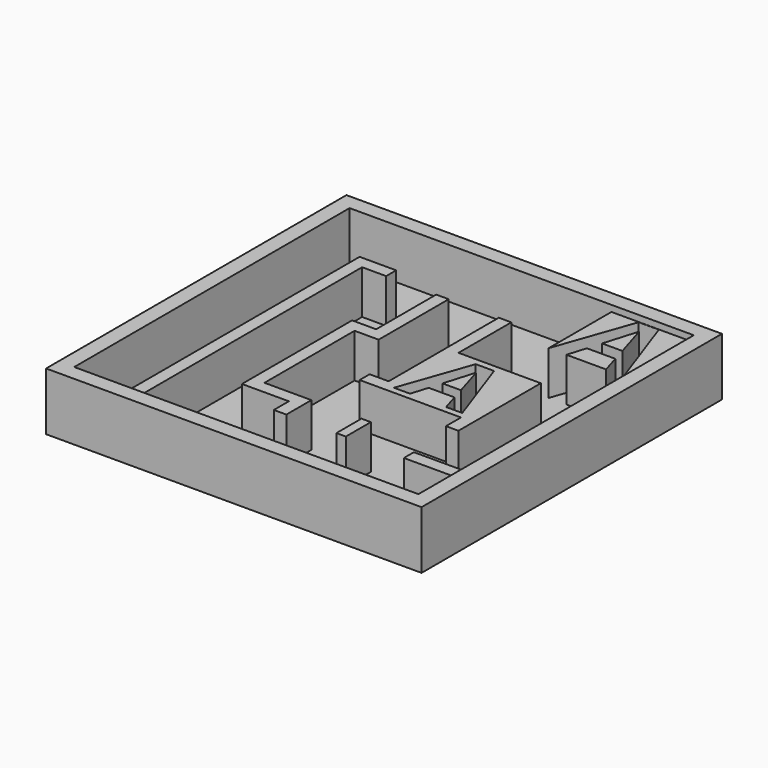
from build123d import *

# Parameters (mm, degrees)
F0_W         = 38.1
F0_H         = 38.1
F1_DEPTH     = 0.79375
F2_W         = 38.1
F2_H         = 38.1
F2_W_2       = 34.925
F2_H_2       = 34.925
F3_DEPTH     = 5.08
F4_W         = 5.5410787107
F4_H         = 1.27
F4_TEXT_SIZE = 11.0670119076
F4_W_2       = 0.9547267341
F4_H_2       = 3.175
F5_DEPTH     = 4.445
F7_DEPTH     = 25.4
F6_R         = 1.27
F6_TEXT_SIZE = 10.0575314688
F8_DEPTH     = 4.445
F9_DEPTH     = 4.445
F10_DEPTH    = 0.396875
F11_DEPTH    = 0.396875


# Not quite as in the source:
# - Text() gives the source's letters only with a copy of the font that has no kerning and outlines rounded to 1/6400 em; it was checked with that copy


with BuildPart() as f1:
    # F0 (on Top) → F1 (new body)
    with BuildSketch(Plane.XY):
        with Locations((0.2368067951, -2.7494172126)):
            Rectangle(F0_W, F0_H)
    extrude(amount=F1_DEPTH)

    # F2 (on face) → F3 (join)
    with BuildSketch(Plane.XY.offset(0.79375)):
        with Locations((0.2368067951, -2.7494172126)):
            Rectangle(F2_W, F2_H)
        with Locations((0.2368067951, -2.7494172126)):
            Rectangle(F2_W_2, F2_H_2, mode=Mode.SUBTRACT)
    extrude(amount=F3_DEPTH)

    # F4 (on face) → F5 (join)
    with BuildSketch(Plane.XY.offset(0.79375)):
        Polygon((-12.1456932049, 9.6330827874), (-12.1456932049, -20.2119172126), (-10.8756932049, -20.2119172126), (-10.8756932049, 8.3630827874), (-8.4345579745, 8.3630827874), (-8.4345579745, 9.6330827874), (-10.8756932049, 9.6330827874), align=None)
        with Locations((14.9287674398, -14.4969172126)):
            Rectangle(F4_W, F4_H)
        Polygon((17.6993067951, 14.7130827874), (9.3454420255, 14.7130827874), (9.3454420255, 6.7448342139), (12.1346748703, 14.6784983752), (14.1820720732, 14.6784983752), (16.9816802417, 6.7448342139), (17.6993067951, 6.7448342139), align=None)
        with Locations((9.3454420255, 6.7448342139)):
            Text('A', F4_TEXT_SIZE, font='Open Sans', font_style=FontStyle.BOLD, text_align=(TextAlign.LEFT, TextAlign.BOTTOM))
        Polygon((11.723120365, 8.6262262382), (11.1507483429, 6.7448342139), (15.1763739243, 6.7448342139), (14.6040019022, 8.6262262382), align=None)
        Polygon((-2.0845579745, 8.3630827874), (-3.3545579745, 8.3630827874), (-3.3545579745, 0.7430827874), (-5.7956932049, 0.7430827874), (-5.7956932049, -0.5269172126), (-5.7956932049, -13.2269172126), (-4.5256932049, -13.2269172126), (-1.035419939, -13.2269172126), (-1.035419939, -15.1319172126), (0.234580061, -15.1319172126), (0.234580061, -13.2269172126), (0.234580061, -11.9569172126), (-4.5256932049, -11.9569172126), (-4.5256932049, -0.5269172126), (-2.0845579745, -0.5269172126), (-2.0845579745, 0.7430827874), align=None)
        Polygon((4.2654420255, 8.3630827874), (2.9954420255, 8.3630827874), (2.9954420255, 4.3662126074), (2.9954420255, 1.6648342139), (2.9954420255, -5.6069172126), (1.0636646766, -5.6069172126), (1.0636646766, -6.8769172126), (2.9954420255, -6.8769172126), (6.2693067951, -6.8769172126), (11.3493067951, -6.8769172126), (11.3493067951, -8.7819172126), (12.6193067951, -8.7819172126), (12.6193067951, -6.8769172126), (12.6193067951, -6.8514254262), (12.6193067951, 1.6648342139), (4.2654420255, 1.6648342139), align=None)
        with Locations((5.7919434281, -13.5444172126)):
            Rectangle(F4_W_2, F4_H_2)
        with BuildLine():
            Line((12.145050194, 10.030353374), (14.2028227205, 10.030353374))
            add(Edge.make_bspline(
                [(14.2028227205, 10.030353374), (13.4091104603, 12.5861414364), (13.3088156649, 12.9216102349)],
                knots=[0, 0, 0, 1, 1, 1], degree=2))
            add(Edge.make_bspline(
                [(13.3088156649, 12.9216102349), (13.2085208695, 13.2570790333), (13.1652903542, 13.4507517417)],
                knots=[0, 0, 0, 1, 1, 1], degree=2))
            add(Edge.make_bspline(
                [(13.1652903542, 13.4507517417), (12.9871806313, 12.7590634975), (12.145050194, 10.030353374)],
                knots=[0, 0, 0, 1, 1, 1], degree=2))
        make_face()
    extrude(amount=F5_DEPTH)

    # F4 (on face) → F7 (cut)
    with BuildSketch(Plane.XY.offset(0.79375)):
        with Locations((9.3454420255, 6.7448342139)):
            Text('A', F4_TEXT_SIZE, font='Open Sans', font_style=FontStyle.BOLD, text_align=(TextAlign.LEFT, TextAlign.BOTTOM))
    extrude(amount=F7_DEPTH, mode=Mode.SUBTRACT)

    # F6 (on face) → F8 (join)
    with BuildSketch(Plane.XY.offset(0.79375)):
        with Locations((-14.6856932049, -16.8305989355)):
            Circle(F6_R)
        with Locations((15.0401042774, -17.6719172126)):
            Circle(F6_R)
        with Locations((4.0114420255, -6.2115884436)):
            Text('A', F6_TEXT_SIZE, font='Open Sans', font_style=FontStyle.BOLD, text_align=(TextAlign.LEFT, TextAlign.BOTTOM))
    extrude(amount=F8_DEPTH)

    # F6 (on face) → F9 (cut)
    with BuildSketch(Plane.XY.offset(0.79375)):
        with Locations((-14.6856932049, -16.8305989355)):
            Circle(F6_R)
        with Locations((15.0401042774, -17.6719172126)):
            Circle(F6_R)
        with Locations((4.0114420255, -6.2115884436)):
            Text('A', F6_TEXT_SIZE, font='Open Sans', font_style=FontStyle.BOLD, text_align=(TextAlign.LEFT, TextAlign.BOTTOM))
    extrude(amount=F9_DEPTH, mode=Mode.SUBTRACT)

    # F6 (on face) → F10 (cut)
    with BuildSketch(Plane.XY.offset(0.79375)):
        with Locations((-14.6856932049, -16.8305989355)):
            Circle(F6_R)
    extrude(amount=-F10_DEPTH, mode=Mode.SUBTRACT)

    # F6 (on face) → F11 (cut)
    with BuildSketch(Plane.XY.offset(0.79375)):
        with Locations((15.0401042774, -17.6719172126)):
            Circle(F6_R)
    extrude(amount=-F11_DEPTH, mode=Mode.SUBTRACT)


solid = f1.part
